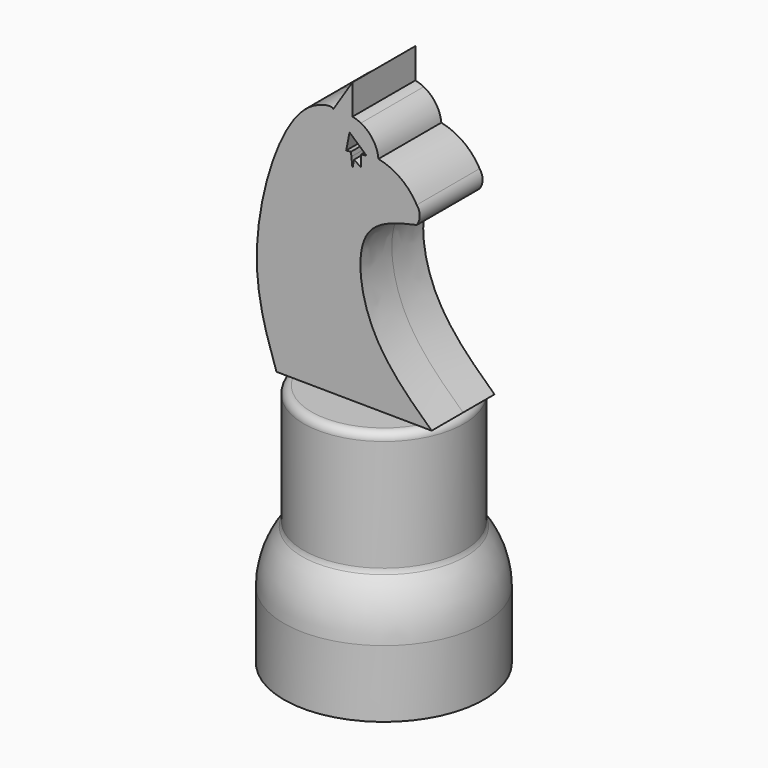
from build123d import *

# Parameters (mm, degrees)
F0_W     = 0.6405061577
F0_H     = 3.9503388107
F3_DEPTH = 1.27
F5_R     = 0.254


# Not quite as in the source:
# - a fillet or chamfer that OpenCascade refuses, or shapes differently, is made with other operations: its cross-section is extruded or revolved along the edge and cut away or added


with BuildPart() as f1:
    # F0 (on Front) → F1 (revolve)
    with BuildSketch(Plane.XZ):
        Polygon((-2.5914753787, -19.5134952664), (0, -19.5134952664), (0, -11.6128176451), (-2.5914753787, -11.6128176451), (-2.5914753787, -15.5631564558), align=None)
        with Locations((-2.9117284575, -17.5383258611)):
            Rectangle(F0_W, F0_H)
    revolve(axis=Axis((0, 0, -15.5631564558), (0, 0, 1)))

    # F4: fillet of radius 2.794 on 1 edges, made by hand

    # F4_s1 → F4_t2 (revolve, cut)
    with BuildSketch(Plane.XZ):
        with BuildLine():
            ThreePointArc((-2.5914753787, -15.5631564558), (-3.0669830384, -16.397365106), (-3.2319815364, -17.3432969758))
            Line((-3.2319815364, -17.3432969758), (-3.2319815364, -15.5631564558))
            Line((-3.2319815364, -15.5631564558), (-2.5914753787, -15.5631564558))
        make_face()
    revolve(axis=Axis((0, 0, -15.5631564558), (0, 0, 1)), mode=Mode.SUBTRACT)

    # F5
    f5_edges = [f1.edges().sort_by_distance(p)[0] for p in [
        (-2.591475, 0, -13.587987),
        (2.591475, 0, -15.563156),
        (2.591475, 0, -11.612818),
    ]]
    fillet(f5_edges, radius=F5_R)


with BuildPart() as f3:
    # F2 (on Front) → F3 (new body, symmetric)
    with BuildSketch(Plane.XZ):
        with BuildLine():
            add(Edge.make_bspline(
                [(-2.4575470015, -11.5132899955), (-2.8040543568, -10.5028159539), (-3.1505617121, -9.4923419122), (-3.0854009092, -8.1228790805)],
                knots=[0, 0, 0, 0, 0.3547843289, 0.3547843289, 0.3547843289, 0.3547843289], degree=3))
            Line((-2.4575470015, -11.5132899955), (2.560271183, -11.5577178076))
            add(Edge.make_bspline(
                [(2.560271183, -11.5577178076), (1.8040367585, -10.8534037399), (0.3574469273, -9.5061316042), (0.0098981732, -6.329177487), (1.4316217442, -6.0063825673), (2.07934645, -5.859320052)],
                knots=[0, 0, 0, 0, 0.3735750804, 0.7146063376, 1, 1, 1, 1], degree=3))
            Line((2.07934645, -5.859320052), (1.7303656682, -5.5492422712))
            Line((1.7303656682, -5.5492422712), (0.4577149879, -4.418461669))
            Line((0.4577149879, -4.418461669), (0.2788823039, -4.4354375079))
            Line((0.2788823039, -4.4354375079), (0.2820669615, -4.8120045103))
            Line((0.2820669615, -4.8120045103), (0.0523033026, -4.6588287686))
            Line((0.0523033026, -4.6588287686), (0, -4.9243257381))
            Line((0, -4.9243257381), (-0.0341830133, -4.6011712362))
            Line((-0.0341830133, -4.6011712362), (-0.0484276129, -4.4665076697))
            Line((-0.0484276129, -4.4665076697), (-0.2024847872, -4.4811316731))
            Line((-0.2024847872, -4.4811316731), (-0.1012423936, -3.9672148204))
            Line((-0.1012423936, -3.9672148204), (-0.0936308252, -3.9285777125))
            Line((-0.0936308252, -3.9285777125), (-0.6285401519, -3.4532979677))
            Line((-0.6285401519, -3.4532979677), (-0.6301807522, -3.4564161403))
            Line((-0.6301807522, -3.4564161403), (-3.0854009092, -8.1228790805))
        make_face()
        with BuildLine():
            add(Edge.make_bspline(
                [(-3.0854009092, -8.1228790805), (-3.009593502, -6.5296601241), (-2.0935214667, -3.5207561612), (-0.6211493091, -3.3432954942), (-0.6258393316, -3.4402559318), (-0.6301807522, -3.4564161403)],
                knots=[0.3547843289, 0.3547843289, 0.3547843289, 0.3547843289, 0.7675367637, 0.9521252582, 0.9860341697, 0.9860341697, 0.9860341697, 0.9860341697], degree=3))
            Line((-3.0854009092, -8.1228790805), (-0.6301807522, -3.4564161403))
        make_face()
        with BuildLine():
            Line((1.7303656682, -5.5492422712), (2.07934645, -5.859320052))
            ThreePointArc((2.07934645, -5.859320052), (2.1746489219, -5.573413102), (2.07934645, -5.2875061519))
            Line((2.07934645, -5.2875061519), (1.7303656682, -5.5492422712))
        make_face()
        Polygon((0, -3.4532979677), (-0.6285401519, -3.4532979677), (-0.0936308252, -3.9285777125), align=None)
        Polygon((0, -2.4760859087), (-0.6285401519, -3.4532979677), (0, -3.4532979677), align=None)
        with BuildLine():
            Line((1.7303656682, -5.5492422712), (2.07934645, -5.2875061519))
            ThreePointArc((2.07934645, -5.2875061519), (1.5590688172, -4.699089309), (0.8404157707, -4.3821334839))
            Line((0.8404157707, -4.3821334839), (0.4577149879, -4.418461669))
            Line((0.4577149879, -4.418461669), (1.7303656682, -5.5492422712))
        make_face()
        with BuildLine():
            Line((0, -3.4532979677), (-0.0936308252, -3.9285777125))
            Line((-0.0936308252, -3.9285777125), (0.1529944372, -4.1477101634))
            Line((0.1529944372, -4.1477101634), (0.2713673383, -3.5468370845))
            ThreePointArc((0.2713673383, -3.5468370845), (0.1389025243, -3.4907292708), (0, -3.4532979677))
        make_face()
        with BuildLine():
            Line((0.4577149879, -4.418461669), (0.8404157707, -4.3821334839))
            ThreePointArc((0.8404157707, -4.3821334839), (0.6632892562, -3.891320245), (0.2713673383, -3.5468370845))
            Line((0.2713673383, -3.5468370845), (0.2773836709, -4.2582329759))
            Line((0.2773836709, -4.2582329759), (0.4577149879, -4.418461669))
        make_face()
        Polygon((0.2713673383, -3.5468370845), (0.1529944372, -4.1477101634), (0.2773836709, -4.2582329759), align=None)
    extrude(amount=F3_DEPTH, both=True)


solid = Compound([f1.part, f3.part])
